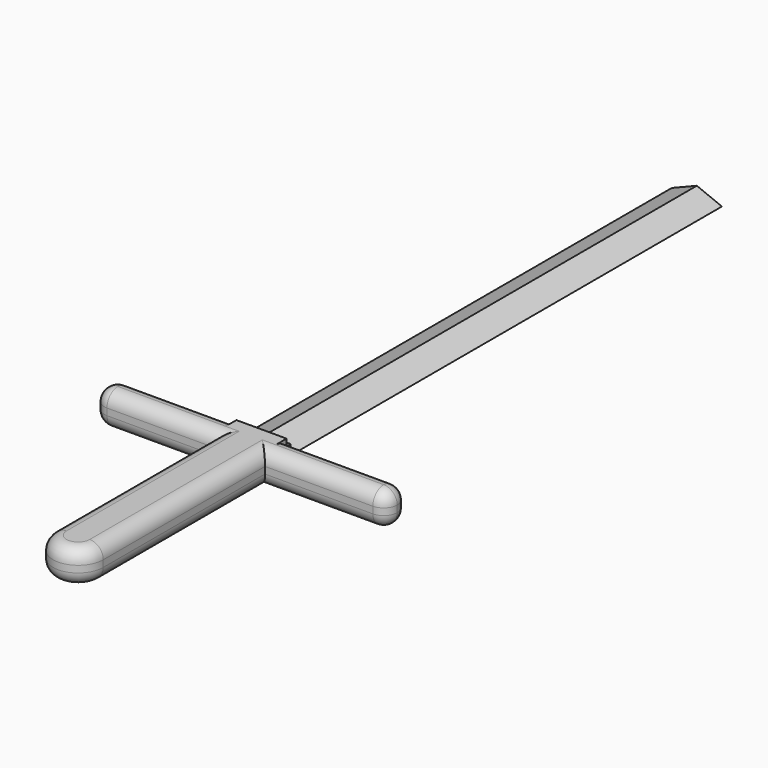
from build123d import *

# Parameters (mm, degrees)
F0_W      = 4.724400118
F0_H      = 62.3315982521
F1_DEPTH  = 6.35
F2_R      = 2.53999
F4_DEPTH  = 1.27
F6_DEPTH  = 1.27
F8_DEPTH  = 25.4
F9_DEPTH  = 50.8
F11_DEPTH = 25.4
F13_DEPTH = 25.4
F15_DEPTH = 101.6


# Not quite as in the source:
# - a fillet or chamfer is up to 0.001 mm smaller than in the source, because OpenCascade refuses the exact size


with BuildPart() as f1:
    # F0 (on Top) → F1 (new body)
    with BuildSketch(Plane.XY):
        with Locations((2.362200059, 31.165799126)):
            Rectangle(F0_W, F0_H)
        with Locations((7.086600177, 31.165799126)):
            Rectangle(F0_W, F0_H)
        Polygon((4.724400118, 75.0454813242), (4.724400118, 62.3315982521), (9.448800236, 62.3315982521), align=None)
        Polygon((4.724400118, 75.0454813242), (0, 62.3315982521), (4.724400118, 62.3315982521), align=None)
        with BuildLine():
            Line((4.724400118, 0), (0, 0))
            Line((0, 0), (-20.32, 0))
            ThreePointArc((-20.32, 0), (-18.5239487758, -0.7439487758), (-17.78, -2.54))
            ThreePointArc((-17.78, -2.54), (-18.5239487758, -4.3360512242), (-20.32, -5.08))
            Line((-20.32, -5.08), (0, -5.08))
            Line((0, -5.08), (9.448800236, -5.08))
            Line((9.448800236, -5.08), (29.768800236, -5.08))
            ThreePointArc((29.768800236, -5.08), (27.228800236, -2.54), (29.768800236, 0))
            Line((29.768800236, 0), (9.448800236, 0))
            Line((9.448800236, 0), (4.724400118, 0))
        make_face()
        with BuildLine():
            Line((9.448800236, -5.08), (0, -5.08))
            Line((0, -5.08), (0, -43.18))
            ThreePointArc((0, -43.18), (4.724400118, -38.455599882), (9.448800236, -43.18))
            Line((9.448800236, -43.18), (9.448800236, -5.08))
        make_face()
        with BuildLine():
            ThreePointArc((-17.78, -2.54), (-18.5239487758, -0.7439487758), (-20.32, 0))
            Line((-20.32, 0), (-20.32, -5.08))
            ThreePointArc((-20.32, -5.08), (-18.5239487758, -4.3360512242), (-17.78, -2.54))
        make_face()
        with BuildLine():
            Line((-20.32, -5.08), (-20.32, 0))
            ThreePointArc((-20.32, 0), (-22.86, -2.54), (-20.32, -5.08))
        make_face()
        with BuildLine():
            Line((29.768800236, -5.08), (29.768800236, 0))
            ThreePointArc((29.768800236, 0), (27.228800236, -2.54), (29.768800236, -5.08))
        make_face()
        with BuildLine():
            ThreePointArc((32.308800236, -2.54), (31.5648514602, -0.7439487758), (29.768800236, 0))
            Line((29.768800236, 0), (29.768800236, -5.08))
            ThreePointArc((29.768800236, -5.08), (31.5648514602, -4.3360512242), (32.308800236, -2.54))
        make_face()
        with BuildLine():
            Line((9.448800236, -43.18), (0, -43.18))
            ThreePointArc((0, -43.18), (4.724400118, -47.904400118), (9.448800236, -43.18))
        make_face()
        with BuildLine():
            ThreePointArc((9.448800236, -43.18), (4.724400118, -38.455599882), (0, -43.18))
            Line((0, -43.18), (9.448800236, -43.18))
        make_face()
    extrude(amount=F1_DEPTH)

    # F2 (radius 2.54 in the source; OpenCascade refuses exactly that, so slightly less here)
    f2_edges = [f1.edges().sort_by_distance(p)[0] for p in [
        (0, -24.13, 6.35),
        (9.4488, -24.13, 6.35),
        (0, -24.13, 0),
        (9.4488, -24.13, 0),
        (19.6088, -5.08, 0),
        (19.6088, 0, 0),
        (-10.16, 0, 0),
        (19.6088, -5.08, 6.35),
        (19.6088, 0, 6.35),
        (-10.16, -5.08, 6.35),
        (-10.16, 0, 6.35),
        (-10.16, -5.08, 0),
    ]]
    fillet(f2_edges, radius=F2_R)

    # F3 (on face) → F4 (cut)
    with BuildSketch(Plane.XY.offset(6.35)):
        Polygon((0, 62.3315982521), (0, 0), (9.448800236, 0), (9.448800236, 62.3315982521), (4.724400118, 75.0454813242), align=None)
    extrude(amount=-F4_DEPTH, mode=Mode.SUBTRACT)

    # F5 (on face) → F6 (cut)
    with BuildSketch(Plane(origin=(0, 0, 0), x_dir=(1, 0, 0), z_dir=(0, 0, -1))):
        Polygon((9.448800236, 0), (0, 0), (0, -62.3315982521), (4.724400118, -75.0454813242), (9.448800236, -62.3315982521), align=None)
    extrude(amount=-F6_DEPTH, mode=Mode.SUBTRACT)

    # F7 (on face) → F8 (cut)
    with BuildSketch(Plane.XY.offset(5.08)):
        Polygon((4.724400118, 75.0454813242), (0, 62.3315982521), (9.448800236, 62.3315982521), align=None)
    extrude(amount=-F8_DEPTH, mode=Mode.SUBTRACT)

    # F9 (add): a face of the model
    f9_faces = [f1.faces().sort_by_distance(p)[0] for p in [
        (4.724400118, 62.3315982521, 3.175),
    ]]
    extrude(f9_faces, amount=F9_DEPTH)

    # F10 (on face) → F11 (cut)
    with BuildSketch(Plane.XY.offset(5.08)):
        Polygon((0, 102.5230064988), (4.724400118, 113.1315982521), (0, 113.1315982521), align=None)
        Polygon((9.448800236, 113.1315982521), (4.724400118, 113.1315982521), (9.448800236, 102.5230064988), align=None)
    extrude(amount=-F11_DEPTH, mode=Mode.SUBTRACT)

    # F12 (on face) → F13 (cut)
    with BuildSketch(Plane.XY.offset(5.08)):
        Polygon((4.724400118, 113.1315982521), (0, 102.5230064988), (9.448800236, 102.5230064988), align=None)
    extrude(amount=-F13_DEPTH, mode=Mode.SUBTRACT)

    # F14 (on face) → F15 (cut)
    with BuildSketch(Plane(origin=(0, 102.5230064988, 0), x_dir=(-1, 0, 0), z_dir=(0, 1, 0))):
        Polygon((0, 5.08), (-4.724400118, 5.08), (0, 3.175), align=None)
        Polygon((0, 1.27), (0, 3.175), (-4.724400118, 1.27), align=None)
        Polygon((-4.724400118, 1.27), (-9.448800236, 3.175), (-9.448800236, 1.27), align=None)
        Polygon((-9.448800236, 3.175), (-4.724400118, 5.08), (-9.448800236, 5.08), align=None)
    extrude(amount=-F15_DEPTH, mode=Mode.SUBTRACT)


solid = f1.part
